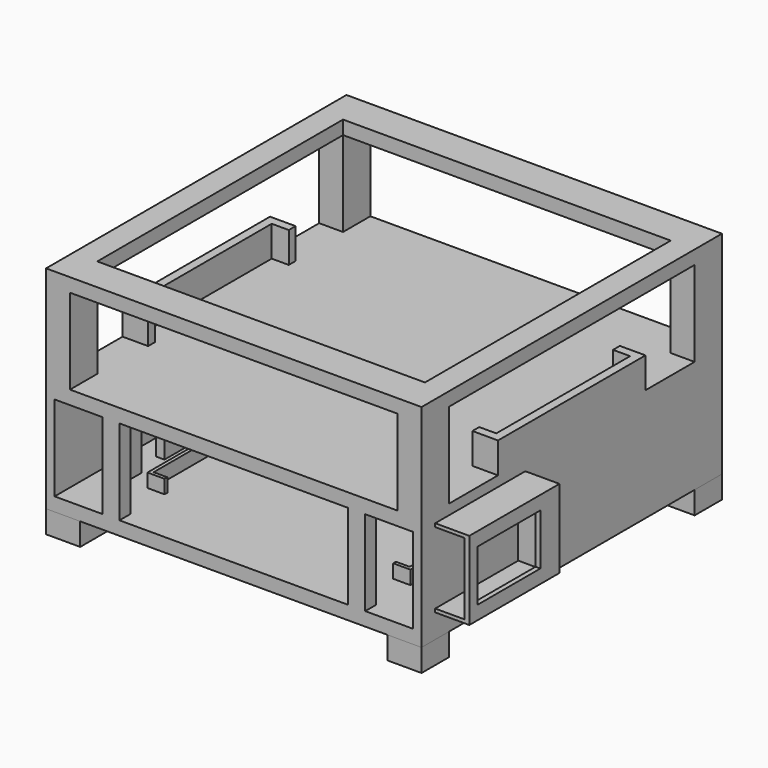
from build123d import *

# Parameters (mm, degrees)
F0_W      = 12.7
F0_H      = 12.7
F1_DEPTH  = 8.382
F2_W      = 139.7
F2_H      = 139.7
F3_DEPTH  = 5.08
F5_W      = 97.79
F5_H      = 97.79
F5_W_2    = 95.25
F5_H_2    = 95.25
F6_DEPTH  = 5.08
F7_W      = 85.09
F7_H      = 139.7
F8_DEPTH  = 5.08
F9_W      = 3.175
F9_H      = 139.7
F9_H_2    = 16.764
F9_H_3    = 12.7
F9_W_2    = 6.35
F9_H_4    = 5.08
F10_DEPTH = 31.75
F11_W     = 139.7
F11_H     = 139.7
F12_DEPTH = 5.08
F13_W     = 139.7
F13_H     = 68.58
F13_W_2   = 133.35
F13_H_2   = 62.23
F14_DEPTH = 11.43
F15_W     = 120.65
F15_H     = 85.1746347484
F16_DEPTH = 25.4
F17_W     = 8.89
F17_H     = 12.7
F18_DEPTH = 31.75
F19_W     = 8.89
F19_H     = 12.7
F19_W_2   = 121.92
F19_H_2   = 114.3
F20_DEPTH = 5.08
F21_W     = 41.91
F21_H     = 29.21
F22_DEPTH = 12.7
F23_W     = 10.922
F23_H     = 26.67
F24_DEPTH = 38.608
F25_W     = 10.922
F25_H     = 6.35
F26_DEPTH = 25.4
F27_W     = 29.21
F27_H     = 19.05
F28_DEPTH = 6.35


# Not quite as in the source:
# - a feature names something its author has since deleted; it is built from what else it names


with BuildPart() as f1:
    # F0 (on Top) → F1 (new body)
    with BuildSketch(Plane.XY):
        with Locations((-63.5, -63.5)):
            Rectangle(F0_W, F0_H)
    extrude(amount=F1_DEPTH)


with BuildPart() as f1b:
    # F0 (on Top) → F1, piece 2 (new body)
    with BuildSketch(Plane.XY):
        with Locations((63.5, -63.5)):
            Rectangle(F0_W, F0_H)
    extrude(amount=F1_DEPTH)


with BuildPart() as f1c:
    # F0 (on Top) → F1, piece 3 (new body)
    with BuildSketch(Plane.XY):
        with Locations((63.5, 63.5)):
            Rectangle(F0_W, F0_H)
    extrude(amount=F1_DEPTH)


with BuildPart() as f1d:
    # F0 (on Top) → F1, piece 4 (new body)
    with BuildSketch(Plane.XY):
        with Locations((-63.5, 63.5)):
            Rectangle(F0_W, F0_H)
    extrude(amount=F1_DEPTH)


with BuildPart() as f3:
    # F2 (on face) → F3 (new body)
    with BuildSketch(Plane.XY.offset(8.382)):
        Rectangle(F2_W, F2_H)
    extrude(amount=F3_DEPTH)

    # F5 (on face) → F6 (join)
    with BuildSketch(Plane.XY.offset(13.462)):
        Rectangle(F5_W, F5_H)
        Rectangle(F5_W_2, F5_H_2, mode=Mode.SUBTRACT)
    extrude(amount=F6_DEPTH)

    # F7 (on face) → F8 (cut)
    with BuildSketch(Plane.XY.offset(13.462)):
        Rectangle(F7_W, F7_H)
    extrude(amount=F8_DEPTH, mode=Mode.SUBTRACT)

    # F9 (on face) → F10 (join)
    with BuildSketch(Plane.XY.offset(13.462)):
        with Locations((-68.2625, 0)):
            Rectangle(F9_W, F9_H)
        with Locations((-57.785, 23.495)):
            Rectangle(F9_W, F9_H_2)
        with Locations((-57.785, 0)):
            Rectangle(F9_W, F9_H_2)
        with Locations((-57.785, -23.495)):
            Rectangle(F9_W, F9_H_2)
        with Locations((-57.785, 48.895)):
            Rectangle(F9_W, F9_H_3)
        with Locations((-57.785, -48.895)):
            Rectangle(F9_W, F9_H_3)
        with Locations((-45.72, 67.31)):
            Rectangle(F9_W_2, F9_H_4)
        with Locations((-45.72, -67.31)):
            Rectangle(F9_W_2, F9_H_4)
        with Locations((57.785, 48.895)):
            Rectangle(F9_W, F9_H_3)
        with Locations((45.72, 67.31)):
            Rectangle(F9_W_2, F9_H_4)
        with Locations((57.785, -48.895)):
            Rectangle(F9_W, F9_H_3)
        with Locations((57.785, 23.495)):
            Rectangle(F9_W, F9_H_2)
        with Locations((45.72, -67.31)):
            Rectangle(F9_W_2, F9_H_4)
        with Locations((57.785, -23.495)):
            Rectangle(F9_W, F9_H_2)
        with Locations((68.2625, 0)):
            Rectangle(F9_W, F9_H)
        with Locations((57.785, 0)):
            Rectangle(F9_W, F9_H_2)
    extrude(amount=F10_DEPTH)

    # F11 (on face) → F12 (join)
    with BuildSketch(Plane.XY.offset(45.212)):
        Rectangle(F11_W, F11_H)
    extrude(amount=F12_DEPTH)

    # F13 (on face) → F14 (join)
    with BuildSketch(Plane.XY.offset(50.292)):
        Rectangle(F13_W, F13_H)
        Rectangle(F13_W_2, F13_H_2, mode=Mode.SUBTRACT)
    extrude(amount=F14_DEPTH)

    # F15 (on face) → F16 (cut)
    with BuildSketch(Plane.XY.offset(50.292)):
        Rectangle(F15_W, F15_H)
    extrude(amount=F16_DEPTH, mode=Mode.SUBTRACT)

    # F17 (on face) → F18 (join)
    with BuildSketch(Plane.XY.offset(50.292)):
        with Locations((-65.405, 63.5)):
            Rectangle(F17_W, F17_H)
        with Locations((65.405, 63.5)):
            Rectangle(F17_W, F17_H)
        with Locations((65.405, -63.5)):
            Rectangle(F17_W, F17_H)
        with Locations((-65.405, -63.5)):
            Rectangle(F17_W, F17_H)
    extrude(amount=F18_DEPTH)

    # F19 (on face) → F20 (join)
    with BuildSketch(Plane.XY.offset(82.042)):
        with Locations((-65.405, -63.5)):
            Rectangle(F19_W, F19_H)
        with Locations((0, -63.5)):
            Rectangle(F19_W_2, F19_H)
        with Locations((-65.405, 0)):
            Rectangle(F19_W, F19_H_2)
        with Locations((65.405, -63.5)):
            Rectangle(F19_W, F19_H)
        with Locations((-65.405, 63.5)):
            Rectangle(F19_W, F19_H)
        with Locations((0, 63.5)):
            Rectangle(F19_W_2, F19_H)
        with Locations((65.405, 0)):
            Rectangle(F19_W, F19_H_2)
        with Locations((65.405, 63.5)):
            Rectangle(F19_W, F19_H)
    extrude(amount=F20_DEPTH)

    # F21 (on face) → F22 (join)
    with BuildSketch(Plane.YZ.offset(69.85)):
        with Locations((-42.545, 31.877)):
            Rectangle(F21_W, F21_H)
    extrude(amount=F22_DEPTH)

    # F23 (on face) → F24 (cut)
    with BuildSketch(Plane.XZ.offset(63.5)):
        with Locations((75.311, 31.877)):
            Rectangle(F23_W, F23_H)
    extrude(amount=-F24_DEPTH, mode=Mode.SUBTRACT)

    # F25 (on face) → F26 (cut)
    with BuildSketch(Plane(origin=(0, -21.59, 0), x_dir=(-1, 0, 0), z_dir=(0, 1, 0))):
        with Locations((-75.311, 42.037)):
            Rectangle(F25_W, F25_H)
    extrude(amount=-F26_DEPTH, mode=Mode.SUBTRACT)

    # F27 (on face) → F28 (cut)
    with BuildSketch(Plane.YZ.offset(82.55)):
        with Locations((-45.085, 31.877)):
            Rectangle(F27_W, F27_H)
    extrude(amount=-F28_DEPTH, mode=Mode.SUBTRACT)


solid = Compound([f1.part, f1b.part, f1c.part, f1d.part, f3.part])
